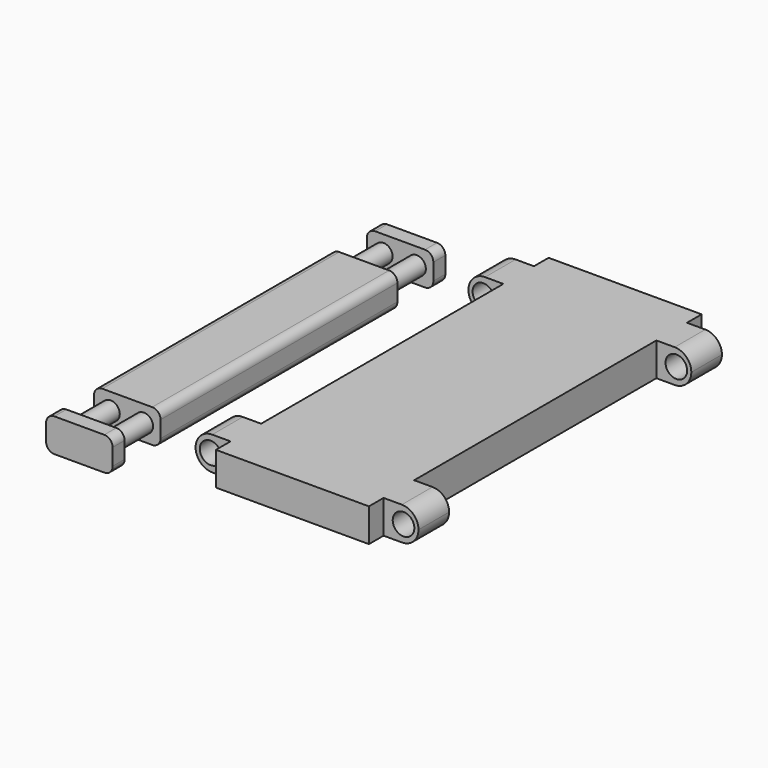
from build123d import *

# Parameters (mm, degrees)
F0_W      = 8
F0_H      = 4
F1_DEPTH  = 25
F2_W      = 8
F2_H      = 5.4
F3_DEPTH  = 25
F4_R      = 1.1
F5_DEPTH  = 7
F6_R      = 1
F8_W      = 9.2
F8_H      = 4
F9_DEPTH  = 25
F10_W     = 4.6
F10_H     = 4
F11_DEPTH = 4.2
F12_R     = 1.3
F13_DEPTH = 25
F14_R     = 1.99999


# Not quite as in the source:
# - a fillet or chamfer is up to 0.001 mm smaller than in the source, because OpenCascade refuses the exact size


with BuildPart() as f1:
    # F0 (on Front) → F1 (new body)
    with BuildSketch(Plane.XZ):
        with Locations((-52.9895666987, 26.7937131725)):
            Rectangle(F0_W, F0_H)
    extrude(amount=F1_DEPTH)

    # F2 (on face) → F3 (cut)
    with BuildSketch(Plane.XY.offset(28.7937131725)):
        with Locations((-52.9895666987, -20.5)):
            Rectangle(F2_W, F2_H)
    extrude(amount=-F3_DEPTH, mode=Mode.SUBTRACT)

    # F4 (on face) → F5 (join)
    with BuildSketch(Plane.XZ.offset(17.8)):
        with Locations((-54.9895666987, 26.7937131725)):
            Circle(F4_R)
        with Locations((-50.9895666987, 26.7937131725)):
            Circle(F4_R)
    extrude(amount=F5_DEPTH)

    # F6
    f6_edges = [f1.edges().sort_by_distance(p)[0] for p in [
        (-56.989567, -8.9, 28.793713),
        (-48.989567, -8.9, 28.793713),
        (-48.989567, -8.9, 24.793713),
        (-48.989567, -24.1, 28.793713),
        (-56.989567, -24.1, 28.793713),
        (-48.989567, -24.1, 24.793713),
        (-56.989567, -8.9, 24.793713),
        (-56.989567, -24.1, 24.793713),
    ]]
    fillet(f6_edges, radius=F6_R)

    # F7: F1 across plane


with BuildPart() as f1_1:
    add(f1.part)
    add(f1.part.mirror(Plane.XZ))


with BuildPart() as f9:
    # F8 (on Front) → F9 (new body)
    with BuildSketch(Plane.XZ):
        with Locations((-22.7743378759, 29.5677930117)):
            Rectangle(F8_W, F8_H)
    extrude(amount=F9_DEPTH)

    # F10 (on face) → F11 (join)
    with BuildSketch(Plane.YZ.offset(-18.1743378759)):
        with Locations((-20.5, 29.5677930117)):
            Rectangle(F10_W, F10_H)
    extrude(amount=F11_DEPTH)

    # F12 (on face) → F13 (cut)
    with BuildSketch(Plane.XZ.offset(22.8)):
        with Locations((-15.7743378759, 29.5677930117)):
            Circle(F12_R)
    extrude(amount=-F13_DEPTH, mode=Mode.SUBTRACT)

    # F14 (radius 2 in the source; OpenCascade refuses exactly that, so slightly less here)
    f14_edges = [f9.edges().sort_by_distance(p)[0] for p in [
        (-13.974338, -20.5, 31.567793),
        (-13.974338, -20.5, 27.567793),
    ]]
    fillet(f14_edges, radius=F14_R)

    # F15: F9 across face


with BuildPart() as f9_1:
    add(f9.part)
    add(f9.part.mirror(Plane(origin=(-27.3743378759, -12.5, 29.5677930117), x_dir=(0, -1, 0), z_dir=(-1, 0, 0))))

    # F16: F9 across face


with BuildPart() as f9_2:
    add(f9_1.part)
    add(f9_1.part.mirror(Plane(origin=(-27.3743378759, 0, 29.5677930117), x_dir=(-1, 0, 0), z_dir=(0, 1, 0))))


solid = Compound([f1_1.part, f9_2.part])
